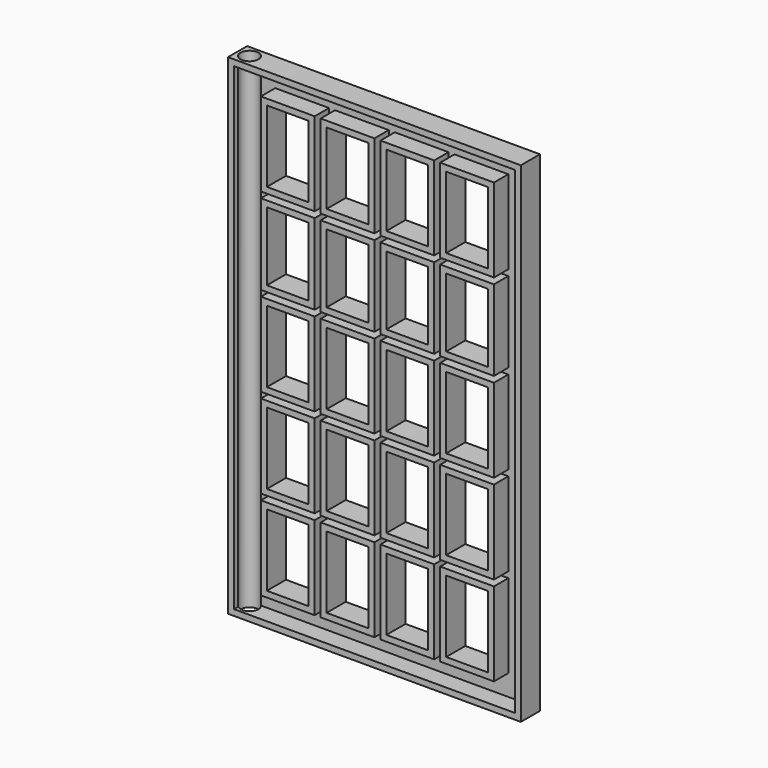
from build123d import *

# Parameters (mm, degrees)
F0_W     = 49
F0_H     = 82
F0_W_2   = 40
F0_H_2   = 74
F0_W_3   = 7
F0_H_3   = 12
F0_H_4   = 11.5
F1_DEPTH = 4
F2_T     = -1
F4_D     = 3


# Not quite as in the source:
# - a feature names something its author has since deleted; it is built from what else it names


with BuildPart() as f1:
    # F0 (on Front) → F1 (new body)
    with BuildSketch(Plane.XZ):
        with Locations((33.611113002, 41)):
            Rectangle(F0_W, F0_H)
        with Locations((34.111113002, 41)):
            Rectangle(F0_W_2, F0_H_2, mode=Mode.SUBTRACT)
        with Locations((34.111113002, 41)):
            Rectangle(F0_W_2, F0_H_2)
        with Locations((19.111113002, 11.5)):
            Rectangle(F0_W_3, F0_H_3, mode=Mode.SUBTRACT)
        with Locations((29.111113002, 11.5)):
            Rectangle(F0_W_3, F0_H_3, mode=Mode.SUBTRACT)
        with Locations((19.111113002, 26.5)):
            Rectangle(F0_W_3, F0_H_3, mode=Mode.SUBTRACT)
        with Locations((29.111113002, 26.5)):
            Rectangle(F0_W_3, F0_H_3, mode=Mode.SUBTRACT)
        with Locations((39.111113002, 11.5)):
            Rectangle(F0_W_3, F0_H_3, mode=Mode.SUBTRACT)
        with Locations((49.111113002, 11.5)):
            Rectangle(F0_W_3, F0_H_3, mode=Mode.SUBTRACT)
        with Locations((39.111113002, 26.5)):
            Rectangle(F0_W_3, F0_H_3, mode=Mode.SUBTRACT)
        with Locations((49.111113002, 26.5)):
            Rectangle(F0_W_3, F0_H_3, mode=Mode.SUBTRACT)
        with Locations((19.111113002, 41.5)):
            Rectangle(F0_W_3, F0_H_3, mode=Mode.SUBTRACT)
        with Locations((19.111113002, 56.25)):
            Rectangle(F0_W_3, F0_H_4, mode=Mode.SUBTRACT)
        with Locations((29.111113002, 41.5)):
            Rectangle(F0_W_3, F0_H_3, mode=Mode.SUBTRACT)
        with Locations((29.111113002, 56.25)):
            Rectangle(F0_W_3, F0_H_4, mode=Mode.SUBTRACT)
        with Locations((19.111113002, 71)):
            Rectangle(F0_W_3, F0_H_3, mode=Mode.SUBTRACT)
        with Locations((29.111113002, 71)):
            Rectangle(F0_W_3, F0_H_3, mode=Mode.SUBTRACT)
        with Locations((39.111113002, 41.5)):
            Rectangle(F0_W_3, F0_H_3, mode=Mode.SUBTRACT)
        with Locations((39.111113002, 56.25)):
            Rectangle(F0_W_3, F0_H_4, mode=Mode.SUBTRACT)
        with Locations((49.111113002, 41.5)):
            Rectangle(F0_W_3, F0_H_3, mode=Mode.SUBTRACT)
        with Locations((49.111113002, 56.25)):
            Rectangle(F0_W_3, F0_H_4, mode=Mode.SUBTRACT)
        with Locations((39.111113002, 71)):
            Rectangle(F0_W_3, F0_H_3, mode=Mode.SUBTRACT)
        with Locations((49.111113002, 71)):
            Rectangle(F0_W_3, F0_H_3, mode=Mode.SUBTRACT)
    extrude(amount=F1_DEPTH)

    # F2
    f2_openings = [f1.faces().sort_by_distance(p)[0] for p in [
        (33.256946, -4, 40.840774),
    ]]
    offset(amount=F2_T, openings=f2_openings, kind=Kind.INTERSECTION)

    # F4 (through all)
    with Locations(Plane(origin=(0, 0, 0), x_dir=(1, 0, 0), z_dir=(0, 0, -1))):
        with Locations((11.111113002, 2)):
            Hole(F4_D / 2)


solid = f1.part
